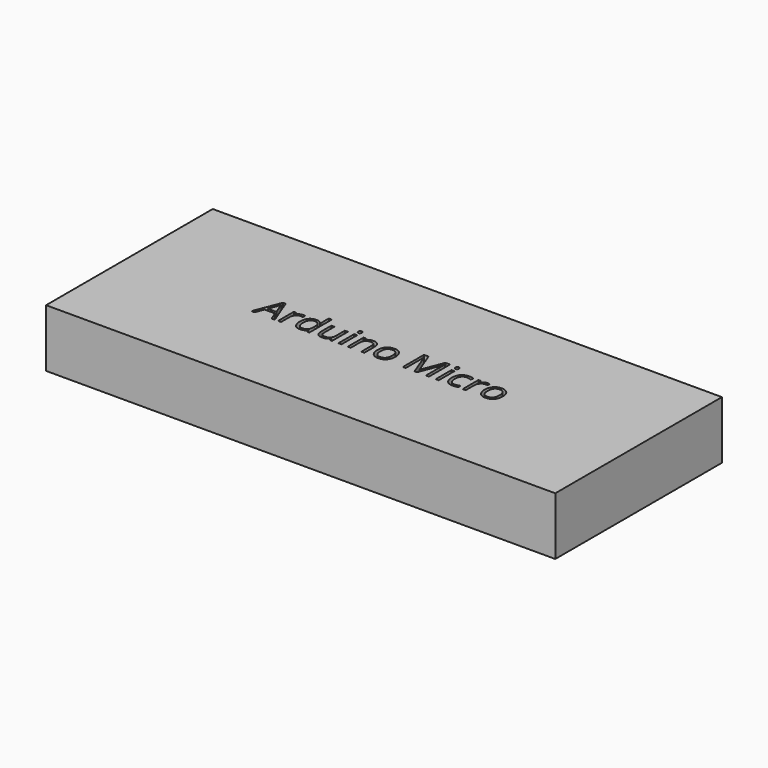
from build123d import *

# Parameters (mm, degrees)
F0_W         = 44
F0_H         = 18
F1_DEPTH     = 5
F2_TEXT_SIZE = 3.1925815468
F3_DEPTH     = 25


# Not quite as in the source:
# - Text() gives the source's letters only with a copy of the font that has no kerning and outlines rounded to 1/6400 em; it was checked with that copy


with BuildPart() as f1:
    # F0 (on Top) → F1 (new body)
    with BuildSketch(Plane.XY):
        Rectangle(F0_W, F0_H)
    extrude(amount=F1_DEPTH)

    # F2 (on face) → F3 (cut)
    with BuildSketch(Plane.XY.offset(5)):
        with Locations((-10.637961328, -1.0182933183)):
            Text('Arduino Micro', F2_TEXT_SIZE, font='Open Sans', text_align=(TextAlign.LEFT, TextAlign.BOTTOM))
    extrude(amount=-F3_DEPTH, mode=Mode.SUBTRACT)


solid = f1.part
